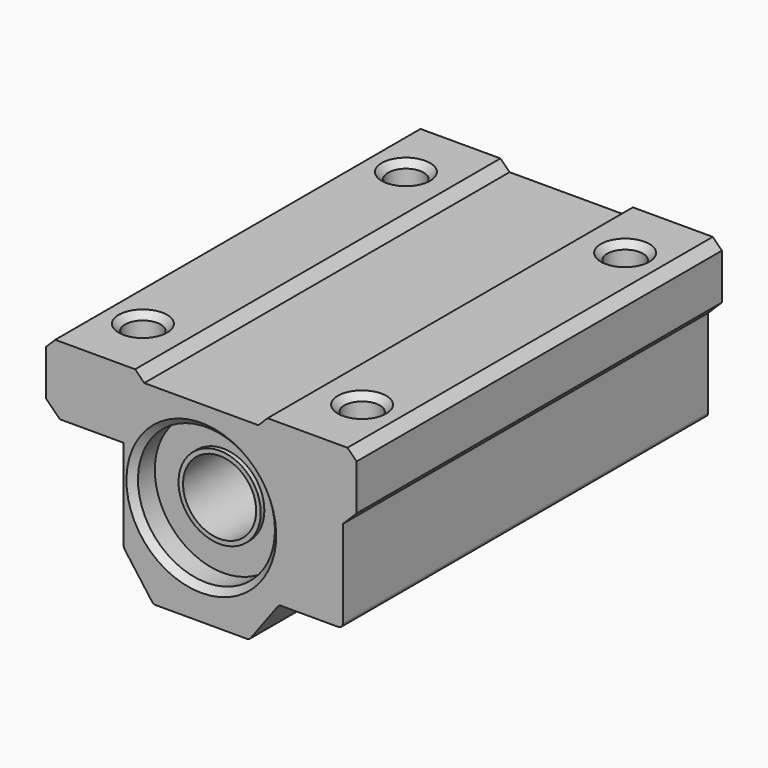
from build123d import *

# Parameters (mm, degrees)
F1_DEPTH       = 25
F2_SIZE        = 0.99999
F3_SIZE        = 1.49999
F4_R           = 0.5
F6_D           = 3.6
F6_CBORE_D     = 3.9
F6_CBORE_DEPTH = 6
F7_SIZE        = 0.7
F0_R           = 4.5
F8_DEPTH       = 22
F0_R_2         = 4
F9_DEPTH       = 22.5


# Not quite as in the source:
# - a fillet or chamfer is up to 0.001 mm smaller than in the source, because OpenCascade refuses the exact size


with BuildPart() as f1:
    # F0 (on Front) → F1 (new body, symmetric)
    with BuildSketch(Plane.XZ):
        with BuildLine():
            ThreePointArc((0, 7.5), (5.3033008589, 5.3033008589), (7.5, 0))
            ThreePointArc((7.5, 0), (5.3033008589, -5.3033008589), (0, -7.5))
            Line((0, -7.5), (0, -11))
            Line((0, -11), (5.25, -11))
            Line((5.25, -11), (8.5, -6.6))
            Line((8.5, -6.6), (15.5, -6.6))
            Line((15.5, -6.6), (15.5, 3.5))
            Line((15.5, 3.5), (17, 3.5))
            Line((17, 3.5), (17, 11))
            Line((17, 11), (7.25, 11))
            Line((7.25, 11), (7.25, 10))
            Line((7.25, 10), (0, 10))
            Line((0, 10), (0, 7.5))
        make_face()
        with BuildLine():
            ThreePointArc((0, -7.5), (-7.5, 0), (0, 7.5))
            Line((0, 7.5), (0, 10))
            Line((0, 10), (-7.25, 10))
            Line((-7.25, 10), (-7.25, 11))
            Line((-7.25, 11), (-17, 11))
            Line((-17, 11), (-17, 3.5))
            Line((-17, 3.5), (-15.5, 3.5))
            Line((-15.5, 3.5), (-8.5, 3.5))
            Line((-8.5, 3.5), (-8.5, -6.6))
            Line((-8.5, -6.6), (-5.25, -11))
            Line((-5.25, -11), (0, -11))
            Line((0, -11), (0, -7.5))
        make_face()
    extrude(amount=F1_DEPTH, both=True)

    # F2 (size 1 in the source; OpenCascade refuses exactly that, so slightly less here)
    f2_edges = [f1.edges().sort_by_distance(p)[0] for p in [
        (7.25, 0, 10),
        (17, 0, 11),
        (-7.25, 0, 10),
        (-17, 0, 11),
    ]]
    chamfer(f2_edges, length=F2_SIZE)

    # F3 (size 1.5 in the source; OpenCascade refuses exactly that, so slightly less here)
    f3_edges = [f1.edges().sort_by_distance(p)[0] for p in [
        (17, 0, 3.5),
        (-17, 0, 3.5),
    ]]
    chamfer(f3_edges, length=F3_SIZE)

    # F4
    f4_edges = [f1.edges().sort_by_distance(p)[0] for p in [
        (15.5, 0, -6.6),
        (8.5, 0, -6.6),
        (5.25, 0, -11),
        (-5.25, 0, -11),
        (-8.5, 0, -6.6),
    ]]
    fillet(f4_edges, radius=F4_R)

    # F6 (through all)
    with Locations(Plane.XY.offset(11)):
        with Locations((12, 18), (12, -18), (-12, 18), (-12, -18)):
            CounterBoreHole(F6_D / 2, F6_CBORE_D / 2, F6_CBORE_DEPTH)

    # F7
    f7_edges = [f1.edges().sort_by_distance(p)[0] for p in [
        (-7.5, -25, 0),
        (-7.5, 25, 0),
        (10.05, 18, 11),
        (10.05, -18, 11),
        (-13.95, 18, 11),
        (-13.95, -18, 11),
    ]]
    chamfer(f7_edges, length=F7_SIZE)


with BuildPart() as f8:
    # F0 (on Front) → F8 (new body, symmetric)
    with BuildSketch(Plane.XZ):
        with BuildLine():
            ThreePointArc((0, -7.5), (5.3033008589, -5.3033008589), (7.5, 0))
            ThreePointArc((7.5, 0), (5.3033008589, 5.3033008589), (0, 7.5))
            ThreePointArc((0, 7.5), (-7.5, 0), (0, -7.5))
        make_face()
        Circle(F0_R, mode=Mode.SUBTRACT)
    extrude(amount=F8_DEPTH, both=True)

    # F0 (on Front) → F9 (join, symmetric)
    with BuildSketch(Plane.XZ):
        Circle(F0_R)
        Circle(F0_R_2, mode=Mode.SUBTRACT)
    extrude(amount=F9_DEPTH, both=True)


solid = Compound([f1.part, f8.part])
